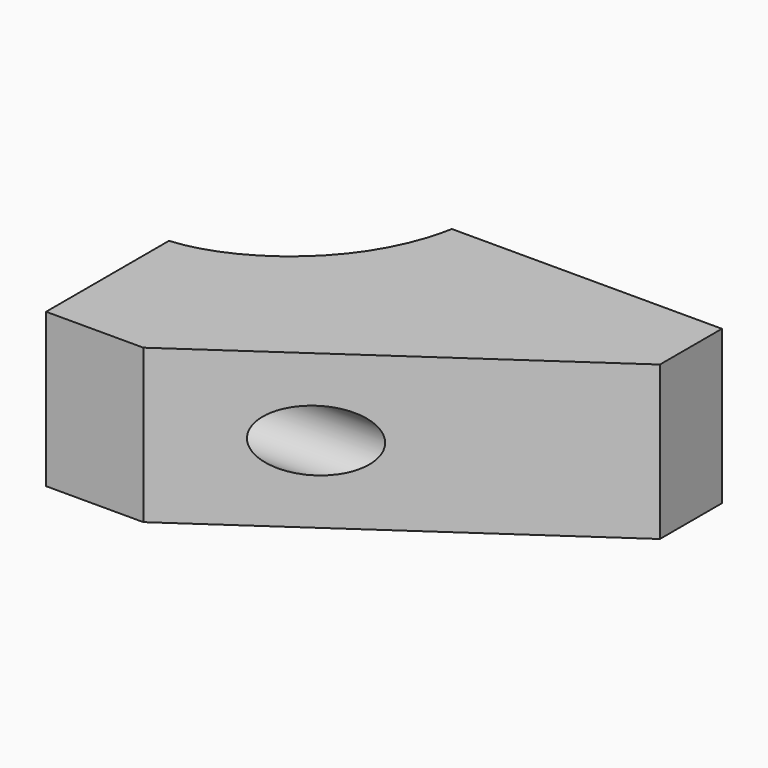
from build123d import *

# Parameters (mm, degrees)
F1_DEPTH = 31.75
F3_D     = 12.7


with BuildPart() as f1:
    # F0 (on Top) → F1 (new body)
    with BuildSketch(Plane.XY):
        with BuildLine():
            Line((45.9964759648, 36.0500998795), (-9.8253758624, 36.0500998795))
            add(Edge.make_bspline(
                [(-42.9035240352, 4.3000998795), (-34.7231067307, 4.914947889), (-18.4671684559, 14.0682512449), (-11.2220877593, 28.5159185869), (-9.8253758624, 36.0500998795)],
                knots=[0, 0, 0, 0, 0.5112036525, 1, 1, 1, 1], degree=3))
            Line((-42.9035240352, 4.3000998795), (-42.9035240352, -27.4499001205))
            Line((-42.9035240352, -27.4499001205), (-22.798109327, -27.4499001205))
            Line((-22.798109327, -27.4499001205), (45.9964759648, 20.0334768742))
            Line((45.9964759648, 20.0334768742), (45.9964759648, 36.0500998795))
        make_face()
    extrude(amount=F1_DEPTH)

    # F3 (through all)
    with Locations(Plane(origin=(-42.9035240352, 0, 0), x_dir=(0, -1, 0), z_dir=(-1, 0, 0))):
        with Locations((11.5749001205, 15.875)):
            Hole(F3_D / 2)


solid = f1.part
